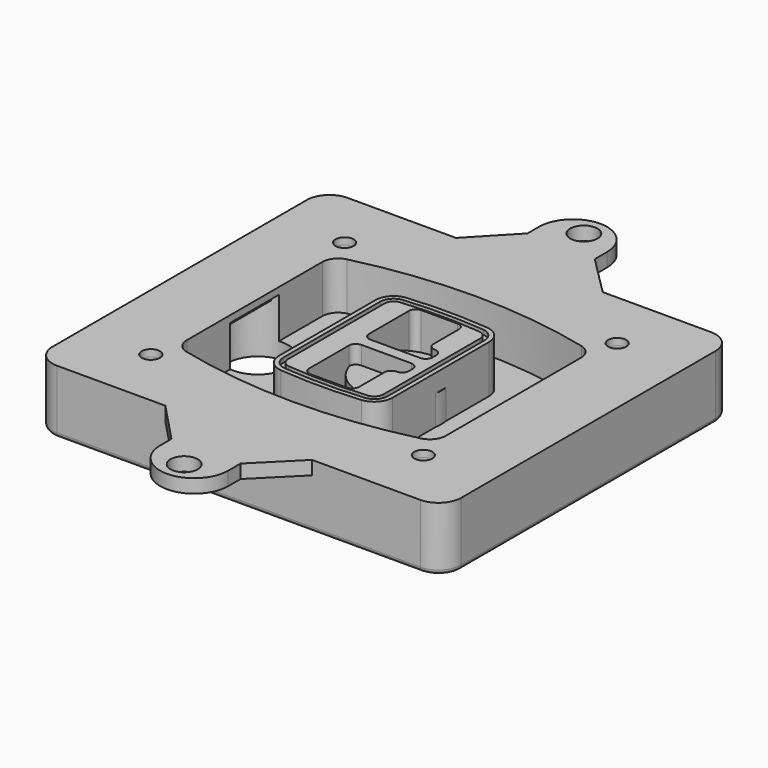
from build123d import *

# Parameters (mm, degrees)
F0_R      = 4
F1_DEPTH  = 25
F2_DEPTH  = 3
F3_DEPTH  = 18
F5_DEPTH  = 21
F6_DEPTH  = 2
F8_DEPTH  = 20
F9_DEPTH  = 16
F10_DEPTH = 25
F7_R      = 6
F7_R_2    = 4
F11_DEPTH = 6
F13_DEPTH = 9
F15_R     = 2
F16_R     = 4
F16_R_2   = 6
F17_DEPTH = 3


# Not quite as in the source:
# - a feature of the source that left no trace in its solid (it failed there, or was rolled back) is left out
# - a feature names something its author has since deleted; it is built from what else it names


with BuildPart() as f1:
    # F0 (on Top) → F1 (new body)
    with BuildSketch(Plane.XY):
        with BuildLine():
            ThreePointArc((-90, -70), (-87.0710678119, -77.0710678119), (-80, -80))
            Line((-80, -80), (80, -80))
            ThreePointArc((80, -80), (87.0710678119, -77.0710678119), (90, -70))
            Line((90, -70), (90, 70))
            ThreePointArc((90, 70), (87.0710678119, 77.0710678119), (80, 80))
            Line((80, 80), (-80, 80))
            ThreePointArc((-80, 80), (-87.0710678119, 77.0710678119), (-90, 70))
            Line((-90, 70), (-90, -70))
        make_face()
        with Locations((-60, -53.3333333333)):
            Circle(F0_R, mode=Mode.SUBTRACT)
        with Locations((60, -53.3333333333)):
            Circle(F0_R, mode=Mode.SUBTRACT)
        with Locations((-60, 53.3333333333)):
            Circle(F0_R, mode=Mode.SUBTRACT)
        with BuildLine():
            ThreePointArc((-64, 37.2990447398), (-61.0143011354, 45.9411029726), (-53.3306899286, 50.8970778549))
            ThreePointArc((-53.3306899286, 50.8970778549), (0, 57.3333333333), (53.3306899286, 50.8970778549))
            ThreePointArc((53.3306899286, 50.8970778549), (61.0143011354, 45.9411029726), (64, 37.2990447398))
            Line((64, 37.2990447398), (64, -37.2990447398))
            ThreePointArc((64, -37.2990447398), (61.0143011354, -45.9411029726), (53.3306899286, -50.8970778549))
            ThreePointArc((53.3306899286, -50.8970778549), (0, -57.3333333333), (-53.3306899286, -50.8970778549))
            ThreePointArc((-53.3306899286, -50.8970778549), (-61.0143011354, -45.9411029726), (-64, -37.2990447398))
            Line((-64, -37.2990447398), (-64, 37.2990447398))
        make_face(mode=Mode.SUBTRACT)
        with Locations((60, 53.3333333333)):
            Circle(F0_R, mode=Mode.SUBTRACT)
        with BuildLine():
            ThreePointArc((53.3306899286, 50.8970778549), (0, 57.3333333333), (-53.3306899286, 50.8970778549))
            ThreePointArc((-53.3306899286, 50.8970778549), (-61.0143011354, 45.9411029726), (-64, 37.2990447398))
            Line((-64, 37.2990447398), (-64, -37.2990447398))
            ThreePointArc((-64, -37.2990447398), (-61.0143011354, -45.9411029726), (-53.3306899286, -50.8970778549))
            ThreePointArc((-53.3306899286, -50.8970778549), (0, -57.3333333333), (53.3306899286, -50.8970778549))
            ThreePointArc((53.3306899286, -50.8970778549), (61.0143011354, -45.9411029726), (64, -37.2990447398))
            Line((64, -37.2990447398), (64, 37.2990447398))
            ThreePointArc((64, 37.2990447398), (61.0143011354, 45.9411029726), (53.3306899286, 50.8970778549))
        make_face()
        with BuildLine():
            Line((-60, -37.2990447398), (-60, 37.2990447398))
            ThreePointArc((-60, 37.2990447398), (-57.8673579538, 43.4719434775), (-52.3790642347, 47.0119255363))
            ThreePointArc((-52.3790642347, 47.0119255363), (0, 53.3333333333), (52.3790642347, 47.0119255363))
            ThreePointArc((52.3790642347, 47.0119255363), (57.8673579538, 43.4719434775), (60, 37.2990447398))
            Line((60, 37.2990447398), (60, -37.2990447398))
            ThreePointArc((60, -37.2990447398), (57.8673579538, -43.4719434775), (52.3790642347, -47.0119255363))
            ThreePointArc((52.3790642347, -47.0119255363), (0, -53.3333333333), (-52.3790642347, -47.0119255363))
            ThreePointArc((-52.3790642347, -47.0119255363), (-57.8673579538, -43.4719434775), (-60, -37.2990447398))
        make_face(mode=Mode.SUBTRACT)
        with BuildLine():
            ThreePointArc((-52.3790642347, 47.0119255363), (-57.8673579538, 43.4719434775), (-60, 37.2990447398))
            Line((-60, 37.2990447398), (-60, -37.2990447398))
            ThreePointArc((-60, -37.2990447398), (-57.8673579538, -43.4719434775), (-52.3790642347, -47.0119255363))
            ThreePointArc((-52.3790642347, -47.0119255363), (0, -53.3333333333), (52.3790642347, -47.0119255363))
            ThreePointArc((52.3790642347, -47.0119255363), (57.8673579538, -43.4719434775), (60, -37.2990447398))
            Line((60, -37.2990447398), (60, 37.2990447398))
            ThreePointArc((60, 37.2990447398), (57.8673579538, 43.4719434775), (52.3790642347, 47.0119255363))
            ThreePointArc((52.3790642347, 47.0119255363), (0, 53.3333333333), (-52.3790642347, 47.0119255363))
        make_face()
        with BuildLine():
            ThreePointArc((51.6653449643, 44.0980612973), (55.5071505677, 41.6200738562), (57, 37.2990447398))
            Line((57, 37.2990447398), (57, -37.2990447398))
            ThreePointArc((57, -37.2990447398), (55.5071505677, -41.6200738562), (51.6653449643, -44.0980612973))
            ThreePointArc((51.6653449643, -44.0980612973), (0, -50.3333333333), (-51.6653449643, -44.0980612973))
            ThreePointArc((-51.6653449643, -44.0980612973), (-55.5071505677, -41.6200738562), (-57, -37.2990447398))
            Line((-57, -37.2990447398), (-57, 37.2990447398))
            ThreePointArc((-57, 37.2990447398), (-55.5071505677, 41.6200738562), (-51.6653449643, 44.0980612973))
            ThreePointArc((-51.6653449643, 44.0980612973), (0, 50.3333333333), (51.6653449643, 44.0980612973))
        make_face(mode=Mode.SUBTRACT)
        with BuildLine():
            Line((57, -37.2990447398), (57, 37.2990447398))
            ThreePointArc((57, 37.2990447398), (55.5071505677, 41.6200738562), (51.6653449643, 44.0980612973))
            ThreePointArc((51.6653449643, 44.0980612973), (0, 50.3333333333), (-51.6653449643, 44.0980612973))
            ThreePointArc((-51.6653449643, 44.0980612973), (-55.5071505677, 41.6200738562), (-57, 37.2990447398))
            Line((-57, 37.2990447398), (-57, -37.2990447398))
            ThreePointArc((-57, -37.2990447398), (-55.5071505677, -41.6200738562), (-51.6653449643, -44.0980612973))
            ThreePointArc((-51.6653449643, -44.0980612973), (0, -50.3333333333), (51.6653449643, -44.0980612973))
            ThreePointArc((51.6653449643, -44.0980612973), (55.5071505677, -41.6200738562), (57, -37.2990447398))
        make_face()
    extrude(amount=-F1_DEPTH)

    # F0 (on Top) → F2 (join)
    with BuildSketch(Plane.XY):
        with BuildLine():
            ThreePointArc((-52.3790642347, 47.0119255363), (-57.8673579538, 43.4719434775), (-60, 37.2990447398))
            Line((-60, 37.2990447398), (-60, -37.2990447398))
            ThreePointArc((-60, -37.2990447398), (-57.8673579538, -43.4719434775), (-52.3790642347, -47.0119255363))
            ThreePointArc((-52.3790642347, -47.0119255363), (0, -53.3333333333), (52.3790642347, -47.0119255363))
            ThreePointArc((52.3790642347, -47.0119255363), (57.8673579538, -43.4719434775), (60, -37.2990447398))
            Line((60, -37.2990447398), (60, 37.2990447398))
            ThreePointArc((60, 37.2990447398), (57.8673579538, 43.4719434775), (52.3790642347, 47.0119255363))
            ThreePointArc((52.3790642347, 47.0119255363), (0, 53.3333333333), (-52.3790642347, 47.0119255363))
        make_face()
        with BuildLine():
            ThreePointArc((51.6653449643, 44.0980612973), (55.5071505677, 41.6200738562), (57, 37.2990447398))
            Line((57, 37.2990447398), (57, -37.2990447398))
            ThreePointArc((57, -37.2990447398), (55.5071505677, -41.6200738562), (51.6653449643, -44.0980612973))
            ThreePointArc((51.6653449643, -44.0980612973), (0, -50.3333333333), (-51.6653449643, -44.0980612973))
            ThreePointArc((-51.6653449643, -44.0980612973), (-55.5071505677, -41.6200738562), (-57, -37.2990447398))
            Line((-57, -37.2990447398), (-57, 37.2990447398))
            ThreePointArc((-57, 37.2990447398), (-55.5071505677, 41.6200738562), (-51.6653449643, 44.0980612973))
            ThreePointArc((-51.6653449643, 44.0980612973), (0, 50.3333333333), (51.6653449643, 44.0980612973))
        make_face(mode=Mode.SUBTRACT)
    extrude(amount=F2_DEPTH)

    # F0 (on Top) → F3 (cut)
    with BuildSketch(Plane.XY):
        with BuildLine():
            Line((57, -37.2990447398), (57, 37.2990447398))
            ThreePointArc((57, 37.2990447398), (55.5071505677, 41.6200738562), (51.6653449643, 44.0980612973))
            ThreePointArc((51.6653449643, 44.0980612973), (0, 50.3333333333), (-51.6653449643, 44.0980612973))
            ThreePointArc((-51.6653449643, 44.0980612973), (-55.5071505677, 41.6200738562), (-57, 37.2990447398))
            Line((-57, 37.2990447398), (-57, -37.2990447398))
            ThreePointArc((-57, -37.2990447398), (-55.5071505677, -41.6200738562), (-51.6653449643, -44.0980612973))
            ThreePointArc((-51.6653449643, -44.0980612973), (0, -50.3333333333), (51.6653449643, -44.0980612973))
            ThreePointArc((51.6653449643, -44.0980612973), (55.5071505677, -41.6200738562), (57, -37.2990447398))
        make_face()
    extrude(amount=-F3_DEPTH, mode=Mode.SUBTRACT)

    # F4 (on face) → F5 (join, through all)
    with BuildSketch(Plane.XY.offset(3)):
        with BuildLine():
            ThreePointArc((-25, -26.587695628), (-22.8992979869, -31.9912392117), (-17.7004291845, -34.5569740744))
            ThreePointArc((-17.7004291845, -34.5569740744), (0, -35.3333333333), (17.7004291845, -34.5569740744))
            ThreePointArc((17.7004291845, -34.5569740744), (22.8992979869, -31.9912392117), (25, -26.587695628))
            Line((25, -26.587695628), (25, 26.587695628))
            ThreePointArc((25, 26.587695628), (22.8992979869, 31.9912392117), (17.7004291845, 34.5569740744))
            ThreePointArc((17.7004291845, 34.5569740744), (0, 35.3333333333), (-17.7004291845, 34.5569740744))
            ThreePointArc((-17.7004291845, 34.5569740744), (-22.8992979869, 31.9912392117), (-25, 26.587695628))
            Line((-25, 26.587695628), (-25, -26.587695628))
        make_face()
        with BuildLine():
            ThreePointArc((17.5253218884, 32.5646544628), (21.4244734902, 30.6403533158), (23, 26.587695628))
            Line((23, 26.587695628), (23, -26.587695628))
            ThreePointArc((23, -26.587695628), (21.4244734902, -30.6403533158), (17.5253218884, -32.5646544628))
            ThreePointArc((17.5253218884, -32.5646544628), (0, -33.3333333333), (-17.5253218884, -32.5646544628))
            ThreePointArc((-17.5253218884, -32.5646544628), (-21.4244734902, -30.6403533158), (-23, -26.587695628))
            Line((-23, -26.587695628), (-23, 26.587695628))
            ThreePointArc((-23, 26.587695628), (-21.4244734902, 30.6403533158), (-17.5253218884, 32.5646544628))
            ThreePointArc((-17.5253218884, 32.5646544628), (0, 33.3333333333), (17.5253218884, 32.5646544628))
        make_face(mode=Mode.SUBTRACT)
        with BuildLine():
            Line((23, -26.587695628), (23, 26.587695628))
            ThreePointArc((23, 26.587695628), (21.4244734902, 30.6403533158), (17.5253218884, 32.5646544628))
            ThreePointArc((17.5253218884, 32.5646544628), (0, 33.3333333333), (-17.5253218884, 32.5646544628))
            ThreePointArc((-17.5253218884, 32.5646544628), (-21.4244734902, 30.6403533158), (-23, 26.587695628))
            Line((-23, 26.587695628), (-23, -26.587695628))
            ThreePointArc((-23, -26.587695628), (-21.4244734902, -30.6403533158), (-17.5253218884, -32.5646544628))
            ThreePointArc((-17.5253218884, -32.5646544628), (0, -33.3333333333), (17.5253218884, -32.5646544628))
            ThreePointArc((17.5253218884, -32.5646544628), (21.4244734902, -30.6403533158), (23, -26.587695628))
        make_face()
        with BuildLine():
            ThreePointArc((17.3502145923, 30.5723348512), (19.9496489934, 29.2894674198), (21, 26.587695628))
            Line((21, 26.587695628), (21, -26.587695628))
            ThreePointArc((21, -26.587695628), (19.9496489934, -29.2894674198), (17.3502145923, -30.5723348512))
            ThreePointArc((17.3502145923, -30.5723348512), (0, -31.3333333333), (-17.3502145923, -30.5723348512))
            ThreePointArc((-17.3502145923, -30.5723348512), (-19.9496489934, -29.2894674198), (-21, -26.587695628))
            Line((-21, -26.587695628), (-21, 26.587695628))
            ThreePointArc((-21, 26.587695628), (-19.9496489934, 29.2894674198), (-17.3502145923, 30.5723348512))
            ThreePointArc((-17.3502145923, 30.5723348512), (0, 31.3333333333), (17.3502145923, 30.5723348512))
        make_face(mode=Mode.SUBTRACT)
        with BuildLine():
            Line((21, -26.587695628), (21, 26.587695628))
            ThreePointArc((21, 26.587695628), (19.9496489934, 29.2894674198), (17.3502145923, 30.5723348512))
            ThreePointArc((17.3502145923, 30.5723348512), (0, 31.3333333333), (-17.3502145923, 30.5723348512))
            ThreePointArc((-17.3502145923, 30.5723348512), (-19.9496489934, 29.2894674198), (-21, 26.587695628))
            Line((-21, 26.587695628), (-21, -26.587695628))
            ThreePointArc((-21, -26.587695628), (-19.9496489934, -29.2894674198), (-17.3502145923, -30.5723348512))
            ThreePointArc((-17.3502145923, -30.5723348512), (0, -31.3333333333), (17.3502145923, -30.5723348512))
            ThreePointArc((17.3502145923, -30.5723348512), (19.9496489934, -29.2894674198), (21, -26.587695628))
        make_face()
        with BuildLine():
            Line((-8, -2.5), (14, -2.5))
            ThreePointArc((14, -2.5), (16.1213203436, -3.3786796564), (17, -5.5))
            Line((17, -5.5), (17, -7.5))
            ThreePointArc((17, -7.5), (16.1213203436, -9.6213203436), (14, -10.5))
            ThreePointArc((14, -10.5), (11.8786796564, -11.3786796564), (11, -13.5))
            Line((11, -13.5), (11, -27.5))
            ThreePointArc((11, -27.5), (10.1213203436, -29.6213203436), (8, -30.5))
            Line((8, -30.5), (-8, -30.5))
            ThreePointArc((-8, -30.5), (-10.1213203436, -29.6213203436), (-11, -27.5))
            Line((-11, -27.5), (-11, -5.5))
            ThreePointArc((-11, -5.5), (-10.1213203436, -3.3786796564), (-8, -2.5))
        make_face(mode=Mode.SUBTRACT)
        with BuildLine():
            ThreePointArc((-8, 2.5), (-10.1213203436, 3.3786796564), (-11, 5.5))
            Line((-11, 5.5), (-11, 27.5))
            ThreePointArc((-11, 27.5), (-10.1213203436, 29.6213203436), (-8, 30.5))
            Line((-8, 30.5), (8, 30.5))
            ThreePointArc((8, 30.5), (10.1213203436, 29.6213203436), (11, 27.5))
            Line((11, 27.5), (11, 13.5))
            ThreePointArc((11, 13.5), (11.8786796564, 11.3786796564), (14, 10.5))
            ThreePointArc((14, 10.5), (16.1213203436, 9.6213203436), (17, 7.5))
            Line((17, 7.5), (17, 5.5))
            ThreePointArc((17, 5.5), (16.1213203436, 3.3786796564), (14, 2.5))
            Line((14, 2.5), (-8, 2.5))
        make_face(mode=Mode.SUBTRACT)
    extrude(amount=-F5_DEPTH)

    # F4 (on face) → F6 (cut)
    with BuildSketch(Plane.XY.offset(3)):
        with BuildLine():
            Line((23, -26.587695628), (23, 26.587695628))
            ThreePointArc((23, 26.587695628), (21.4244734902, 30.6403533158), (17.5253218884, 32.5646544628))
            ThreePointArc((17.5253218884, 32.5646544628), (0, 33.3333333333), (-17.5253218884, 32.5646544628))
            ThreePointArc((-17.5253218884, 32.5646544628), (-21.4244734902, 30.6403533158), (-23, 26.587695628))
            Line((-23, 26.587695628), (-23, -26.587695628))
            ThreePointArc((-23, -26.587695628), (-21.4244734902, -30.6403533158), (-17.5253218884, -32.5646544628))
            ThreePointArc((-17.5253218884, -32.5646544628), (0, -33.3333333333), (17.5253218884, -32.5646544628))
            ThreePointArc((17.5253218884, -32.5646544628), (21.4244734902, -30.6403533158), (23, -26.587695628))
        make_face()
        with BuildLine():
            ThreePointArc((17.3502145923, 30.5723348512), (19.9496489934, 29.2894674198), (21, 26.587695628))
            Line((21, 26.587695628), (21, -26.587695628))
            ThreePointArc((21, -26.587695628), (19.9496489934, -29.2894674198), (17.3502145923, -30.5723348512))
            ThreePointArc((17.3502145923, -30.5723348512), (0, -31.3333333333), (-17.3502145923, -30.5723348512))
            ThreePointArc((-17.3502145923, -30.5723348512), (-19.9496489934, -29.2894674198), (-21, -26.587695628))
            Line((-21, -26.587695628), (-21, 26.587695628))
            ThreePointArc((-21, 26.587695628), (-19.9496489934, 29.2894674198), (-17.3502145923, 30.5723348512))
            ThreePointArc((-17.3502145923, 30.5723348512), (0, 31.3333333333), (17.3502145923, 30.5723348512))
        make_face(mode=Mode.SUBTRACT)
    extrude(amount=-F6_DEPTH, mode=Mode.SUBTRACT)

    # F7 (on face) → F8 (join)
    with BuildSketch(Plane(origin=(0, 0, -25), x_dir=(1, 0, 0), z_dir=(0, 0, -1))):
        with BuildLine():
            ThreePointArc((-6.71157564, 0), (6.7567035675, 13.4682792075), (20.224982775, 0))
            Line((20.224982775, 0), (25.224982775, 0))
            ThreePointArc((25.224982775, 0), (6.7567035675, 18.4682792075), (-11.71157564, 0))
            Line((-11.71157564, 0), (-6.71157564, 0))
        make_face()
        with BuildLine():
            Line((-6.71157564, 0), (20.224982775, 0))
            ThreePointArc((20.224982775, 0), (6.7567035675, 13.4682792075), (-6.71157564, 0))
        make_face()
        with BuildLine():
            ThreePointArc((-6.71157564, 0), (6.7567035675, -13.4682792075), (20.224982775, 0))
            Line((20.224982775, 0), (-6.71157564, 0))
        make_face()
        with BuildLine():
            Line((25.224982775, 0), (20.224982775, 0))
            ThreePointArc((20.224982775, 0), (6.7567035675, -13.4682792075), (-6.71157564, 0))
            Line((-6.71157564, 0), (-11.71157564, 0))
            ThreePointArc((-11.71157564, 0), (6.7567035675, -18.4682792075), (25.224982775, 0))
        make_face()
    extrude(amount=-F8_DEPTH)

    # F7 (on face) → F9 (cut)
    with BuildSketch(Plane(origin=(0, 0, -25), x_dir=(1, 0, 0), z_dir=(0, 0, -1))):
        with BuildLine():
            Line((-6.71157564, 0), (20.224982775, 0))
            ThreePointArc((20.224982775, 0), (6.7567035675, 13.4682792075), (-6.71157564, 0))
        make_face()
        with BuildLine():
            ThreePointArc((-6.71157564, 0), (6.7567035675, -13.4682792075), (20.224982775, 0))
            Line((20.224982775, 0), (-6.71157564, 0))
        make_face()
    extrude(amount=-F9_DEPTH, mode=Mode.SUBTRACT)

    # F7 (on face) → F10 (cut)
    with BuildSketch(Plane(origin=(0, 0, -25), x_dir=(1, 0, 0), z_dir=(0, 0, -1))):
        with BuildLine():
            Line((-69.0318229325, 0), (-42.0952645175, 0))
            ThreePointArc((-42.0952645175, 0), (-55.563543725, 13.4682792075), (-69.0318229325, 0))
        make_face()
        with BuildLine():
            ThreePointArc((-69.0318229325, 0), (-55.563543725, -13.4682792075), (-42.0952645175, 0))
            Line((-42.0952645175, 0), (-69.0318229325, 0))
        make_face()
    extrude(amount=-F10_DEPTH, mode=Mode.SUBTRACT)

    # F7 (on face) → F11 (cut)
    with BuildSketch(Plane(origin=(0, 0, -25), x_dir=(1, 0, 0), z_dir=(0, 0, -1))):
        with Locations((60, -53.3333333333)):
            Circle(F7_R)
        with Locations((60, -53.3333333333)):
            Circle(F7_R_2, mode=Mode.SUBTRACT)
        with Locations((-60, -53.3333333333)):
            Circle(F7_R)
        with Locations((-60, -53.3333333333)):
            Circle(F7_R_2, mode=Mode.SUBTRACT)
        with Locations((-60, 53.3333333333)):
            Circle(F7_R)
        with Locations((-60, 53.3333333333)):
            Circle(F7_R_2, mode=Mode.SUBTRACT)
        with Locations((60, 53.3333333333)):
            Circle(F7_R)
        with Locations((60, 53.3333333333)):
            Circle(F7_R_2, mode=Mode.SUBTRACT)
    extrude(amount=-F11_DEPTH, mode=Mode.SUBTRACT)

    # F12 (on face) → F13 (cut, through all)
    with BuildSketch(Plane(origin=(0, 0, -9), x_dir=(1, 0, 0), z_dir=(0, 0, -1))):
        with BuildLine():
            ThreePointArc((20.224982775, 0), (20.1663399806, 1.2554664788), (19.9909222755, 2.5))
            Line((19.9909222755, 2.5), (14, 2.5))
            ThreePointArc((14, 2.5), (16.1213203436, 3.3786796564), (17, 5.5))
            Line((17, 5.5), (17, 7.5))
            ThreePointArc((17, 7.5), (16.1213203436, 9.6213203436), (14, 10.5))
            ThreePointArc((14, 10.5), (12.1627255951, 11.1284134507), (11.0951631559, 12.750384826))
            ThreePointArc((11.0951631559, 12.750384826), (11.0476113807, 12.7664660322), (11, 12.7823698976))
            Line((11, 12.7823698976), (11, -12.7823698976))
            ThreePointArc((11, -12.7823698976), (11.0476113807, -12.7664660322), (11.0951631559, -12.750384826))
            ThreePointArc((11.0951631559, -12.750384826), (12.1627255951, -11.1284134507), (14, -10.5))
            ThreePointArc((14, -10.5), (16.1213203436, -9.6213203436), (17, -7.5))
            Line((17, -7.5), (17, -5.5))
            ThreePointArc((17, -5.5), (16.1213203436, -3.3786796564), (14, -2.5))
            Line((14, -2.5), (19.9909222755, -2.5))
            ThreePointArc((19.9909222755, -2.5), (20.1663399806, -1.2554664788), (20.224982775, 0))
        make_face()
    extrude(amount=F13_DEPTH, mode=Mode.SUBTRACT)

    # F15
    f15_edges = [f1.edges().sort_by_distance(p)[0] for p in [
        (0, -80, -25),
        (-87.071068, -77.071068, -25),
        (-90, 0, -25),
        (-87.071068, 77.071068, -25),
        (87.071068, -77.071068, -25),
        (0, 80, -25),
        (90, 0, -25),
        (87.071068, 77.071068, -25),
    ]]
    fillet(f15_edges, radius=F15_R)

    # F16 (on face) → F17 (join, symmetric)
    with BuildSketch(Plane.XY):
        with BuildLine():
            Line((-32.2853401303, 80), (-80, 80))
            ThreePointArc((-80, 80), (-87.0710678119, 77.0710678119), (-90, 70))
            Line((-90, 70), (-90, -70))
            ThreePointArc((-90, -70), (-87.0710678119, -77.0710678119), (-80, -80))
            Line((-80, -80), (-32.2853401303, -80))
            Line((-32.2853401303, -80), (32.2935394943, -80))
            Line((32.2935394943, -80), (80, -80))
            ThreePointArc((80, -80), (87.0710678119, -77.0710678119), (90, -70))
            Line((90, -70), (90, 70))
            ThreePointArc((90, 70), (87.0710678119, 77.0710678119), (80, 80))
            Line((80, 80), (32.2935394943, 80))
            Line((32.2935394943, 80), (-32.2853401303, 80))
        make_face()
        with Locations((-60, -53.3333333333)):
            Circle(F16_R, mode=Mode.SUBTRACT)
        with Locations((60, -53.3333333333)):
            Circle(F16_R, mode=Mode.SUBTRACT)
        with Locations((-60, 53.3333333333)):
            Circle(F16_R, mode=Mode.SUBTRACT)
        with BuildLine():
            ThreePointArc((60, -37.2990447398), (57.8673579538, -43.4719434775), (52.3790642347, -47.0119255363))
            ThreePointArc((52.3790642347, -47.0119255363), (0, -53.3333333333), (-52.3790642347, -47.0119255363))
            ThreePointArc((-52.3790642347, -47.0119255363), (-57.8673579538, -43.4719434775), (-60, -37.2990447398))
            Line((-60, -37.2990447398), (-60, 37.2990447398))
            ThreePointArc((-60, 37.2990447398), (-57.8673579538, 43.4719434775), (-52.3790642347, 47.0119255363))
            ThreePointArc((-52.3790642347, 47.0119255363), (0, 53.3333333333), (52.3790642347, 47.0119255363))
            ThreePointArc((52.3790642347, 47.0119255363), (57.8673579538, 43.4719434775), (60, 37.2990447398))
            Line((60, 37.2990447398), (60, -37.2990447398))
        make_face(mode=Mode.SUBTRACT)
        with Locations((60, 53.3333333333)):
            Circle(F16_R, mode=Mode.SUBTRACT)
        with BuildLine():
            Line((-15.1811785544, 98), (-32.2853401303, 80))
            Line((-32.2853401303, 80), (32.2935394943, 80))
            Line((32.2935394943, 80), (14.8188214456, 97.4747180487))
            Line((14.8188214456, 97.4747180487), (14.8188214456, 104.25))
            ThreePointArc((14.8188214456, 104.25), (-0.1811785544, 119.25), (-15.1811785544, 104.25))
            Line((-15.1811785544, 104.25), (-15.1811785544, 98))
        make_face()
        with Locations((0, 110)):
            Circle(F16_R_2, mode=Mode.SUBTRACT)
        with BuildLine():
            Line((32.2935394943, -80), (-32.2853401303, -80))
            Line((-32.2853401303, -80), (-15.1811785544, -98))
            Line((-15.1811785544, -98), (-15.1811785544, -104.25))
            ThreePointArc((-15.1811785544, -104.25), (-0.1811785544, -119.25), (14.8188214456, -104.25))
            Line((14.8188214456, -104.25), (14.8188214456, -97.4747180487))
            Line((14.8188214456, -97.4747180487), (32.2935394943, -80))
        make_face()
        with Locations((0, -110)):
            Circle(F16_R_2, mode=Mode.SUBTRACT)
    extrude(amount=F17_DEPTH, both=True)


solid = f1.part
